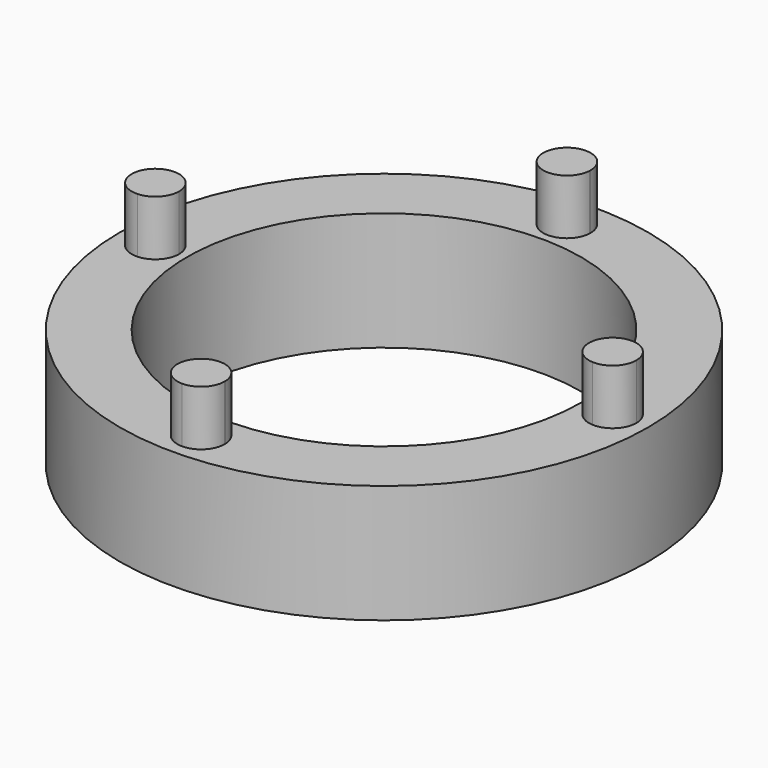
from build123d import *

# Parameters (mm, degrees)
F1_DEPTH = 8.89
F0_R     = 42.545
F0_R_2   = 31.75
F2_DEPTH = 19.05


with BuildPart() as f1:
    # F0 (on Top) → F1 (new body)
    with BuildSketch(Plane.XY):
        with BuildLine():
            ThreePointArc((3.81, 36.83), (2.6940768363, 39.5240768363), (0, 40.64))
            ThreePointArc((0, 40.64), (-2.7628728489, 39.4534773909), (-3.8048999754, 36.6329310345))
            ThreePointArc((-3.8048999754, 36.6329310345), (0, 36.83), (3.8048999754, 36.6329310345))
            ThreePointArc((3.8048999754, 36.6329310345), (3.8087247804, 36.7314325264), (3.81, 36.83))
        make_face()
        with BuildLine():
            ThreePointArc((3.8048999754, 36.6329310345), (0, 36.83), (-3.8048999754, 36.6329310345))
            ThreePointArc((-3.8048999754, 36.6329310345), (0, 33.02), (3.8048999754, 36.6329310345))
        make_face()
    extrude(amount=F1_DEPTH)


with BuildPart() as f1b:
    # F0 (on Top) → F1, piece 2 (new body)
    with BuildSketch(Plane.XY):
        with BuildLine():
            ThreePointArc((-33.02, 0), (-34.0671271511, 2.6234773909), (-36.6329310345, 3.8048999754))
            ThreePointArc((-36.6329310345, 3.8048999754), (-36.83, 0), (-36.6329310345, -3.8048999754))
            ThreePointArc((-36.6329310345, -3.8048999754), (-34.0671271511, -2.6234773909), (-33.02, 0))
        make_face()
        with BuildLine():
            ThreePointArc((-36.6329310345, 3.8048999754), (-39.4534773924, 2.7628728475), (-40.64, -4.1e-09))
            ThreePointArc((-40.64, -4.1e-09), (-39.4534773894, -2.7628728503), (-36.6329310345, -3.8048999754))
            ThreePointArc((-36.6329310345, -3.8048999754), (-36.83, 0), (-36.6329310345, 3.8048999754))
        make_face()
    extrude(amount=F1_DEPTH)


with BuildPart() as f1c:
    # F0 (on Top) → F1, piece 3 (new body)
    with BuildSketch(Plane.XY):
        with BuildLine():
            ThreePointArc((36.83, 0), (36.7806997622, 1.905), (36.6329310345, 3.8048999754))
            ThreePointArc((36.6329310345, 3.8048999754), (33.02, 0), (36.6329310345, -3.8048999754))
            ThreePointArc((36.6329310345, -3.8048999754), (36.7806997622, -1.905), (36.83, 0))
        make_face()
        with BuildLine():
            ThreePointArc((36.6329310345, -3.8048999754), (39.4534773909, -2.7628728489), (40.64, 0))
            ThreePointArc((40.64, 0), (39.4534773909, 2.7628728489), (36.6329310345, 3.8048999754))
            ThreePointArc((36.6329310345, 3.8048999754), (36.7806997622, 1.905), (36.83, 0))
            ThreePointArc((36.83, 0), (36.7806997622, -1.905), (36.6329310345, -3.8048999754))
        make_face()
    extrude(amount=F1_DEPTH)


with BuildPart() as f1d:
    # F0 (on Top) → F1, piece 4 (new body)
    with BuildSketch(Plane.XY):
        with BuildLine():
            ThreePointArc((3.8048999754, -36.6329310345), (0, -33.02), (-3.8048999754, -36.6329310345))
            ThreePointArc((-3.8048999754, -36.6329310345), (0, -36.83), (3.8048999754, -36.6329310345))
        make_face()
        with BuildLine():
            ThreePointArc((-3.8048999754, -36.6329310345), (-2.7628728415, -39.4534773987), (2.15e-08, -40.64))
            ThreePointArc((2.15e-08, -40.64), (2.6940768439, -39.5240768287), (3.81, -36.83))
            ThreePointArc((3.81, -36.83), (3.8087247804, -36.7314325264), (3.8048999754, -36.6329310345))
            ThreePointArc((3.8048999754, -36.6329310345), (0, -36.83), (-3.8048999754, -36.6329310345))
        make_face()
    extrude(amount=F1_DEPTH)


with BuildPart() as f2:
    # F0 (on Top) → F2 (new body)
    with BuildSketch(Plane.XY):
        Circle(F0_R)
        with BuildLine():
            ThreePointArc((0, 40.64), (28.7368195874, 28.7368195874), (40.64, 0))
            ThreePointArc((40.64, 0), (28.736819595, -28.7368195798), (2.15e-08, -40.64))
            ThreePointArc((2.15e-08, -40.64), (-28.7368195784, -28.7368195965), (-40.64, -4.1e-09))
            ThreePointArc((-40.64, -4.1e-09), (-28.7368195889, 28.736819586), (0, 40.64))
        make_face(mode=Mode.SUBTRACT)
        with BuildLine():
            ThreePointArc((36.6329310345, -3.8048999754), (33.02, 0), (36.6329310345, 3.8048999754))
            ThreePointArc((36.6329310345, 3.8048999754), (26.0427427511, 26.0427427511), (3.8048999754, 36.6329310345))
            ThreePointArc((3.8048999754, 36.6329310345), (0, 33.02), (-3.8048999754, 36.6329310345))
            ThreePointArc((-3.8048999754, 36.6329310345), (-26.0427427511, 26.0427427511), (-36.6329310345, 3.8048999754))
            ThreePointArc((-36.6329310345, 3.8048999754), (-34.0671271511, 2.6234773909), (-33.02, 0))
            ThreePointArc((-33.02, 0), (-34.0671271511, -2.6234773909), (-36.6329310345, -3.8048999754))
            ThreePointArc((-36.6329310345, -3.8048999754), (-26.0427427511, -26.0427427511), (-3.8048999754, -36.6329310345))
            ThreePointArc((-3.8048999754, -36.6329310345), (0, -33.02), (3.8048999754, -36.6329310345))
            ThreePointArc((3.8048999754, -36.6329310345), (26.0427427511, -26.0427427511), (36.6329310345, -3.8048999754))
        make_face()
        Circle(F0_R_2, mode=Mode.SUBTRACT)
        with BuildLine():
            ThreePointArc((36.6329310345, 3.8048999754), (39.4534773909, 2.7628728489), (40.64, 0))
            ThreePointArc((40.64, 0), (28.7368195874, 28.7368195874), (0, 40.64))
            ThreePointArc((0, 40.64), (2.6940768363, 39.5240768363), (3.81, 36.83))
            ThreePointArc((3.81, 36.83), (3.8087247804, 36.7314325264), (3.8048999754, 36.6329310345))
            ThreePointArc((3.8048999754, 36.6329310345), (26.0427427511, 26.0427427511), (36.6329310345, 3.8048999754))
        make_face()
        with BuildLine():
            ThreePointArc((2.15e-08, -40.64), (28.736819595, -28.7368195798), (40.64, 0))
            ThreePointArc((40.64, 0), (39.4534773909, -2.7628728489), (36.6329310345, -3.8048999754))
            ThreePointArc((36.6329310345, -3.8048999754), (26.0427427511, -26.0427427511), (3.8048999754, -36.6329310345))
            ThreePointArc((3.8048999754, -36.6329310345), (3.8087247804, -36.7314325264), (3.81, -36.83))
            ThreePointArc((3.81, -36.83), (2.6940768439, -39.5240768287), (2.15e-08, -40.64))
        make_face()
        with BuildLine():
            ThreePointArc((-3.8048999754, 36.6329310345), (-2.7628728489, 39.4534773909), (0, 40.64))
            ThreePointArc((0, 40.64), (-28.7368195889, 28.736819586), (-40.64, -4.1e-09))
            ThreePointArc((-40.64, -4.1e-09), (-39.4534773924, 2.7628728475), (-36.6329310345, 3.8048999754))
            ThreePointArc((-36.6329310345, 3.8048999754), (-26.0427427511, 26.0427427511), (-3.8048999754, 36.6329310345))
        make_face()
        with BuildLine():
            ThreePointArc((-40.64, -4.1e-09), (-28.7368195784, -28.7368195965), (2.15e-08, -40.64))
            ThreePointArc((2.15e-08, -40.64), (-2.7628728415, -39.4534773987), (-3.8048999754, -36.6329310345))
            ThreePointArc((-3.8048999754, -36.6329310345), (-26.0427427511, -26.0427427511), (-36.6329310345, -3.8048999754))
            ThreePointArc((-36.6329310345, -3.8048999754), (-39.4534773894, -2.7628728503), (-40.64, -4.1e-09))
        make_face()
        with BuildLine():
            ThreePointArc((36.6329310345, -3.8048999754), (39.4534773909, -2.7628728489), (40.64, 0))
            ThreePointArc((40.64, 0), (39.4534773909, 2.7628728489), (36.6329310345, 3.8048999754))
            ThreePointArc((36.6329310345, 3.8048999754), (36.7806997622, 1.905), (36.83, 0))
            ThreePointArc((36.83, 0), (36.7806997622, -1.905), (36.6329310345, -3.8048999754))
        make_face()
        with BuildLine():
            ThreePointArc((3.81, 36.83), (2.6940768363, 39.5240768363), (0, 40.64))
            ThreePointArc((0, 40.64), (-2.7628728489, 39.4534773909), (-3.8048999754, 36.6329310345))
            ThreePointArc((-3.8048999754, 36.6329310345), (0, 36.83), (3.8048999754, 36.6329310345))
            ThreePointArc((3.8048999754, 36.6329310345), (3.8087247804, 36.7314325264), (3.81, 36.83))
        make_face()
        with BuildLine():
            ThreePointArc((-3.8048999754, -36.6329310345), (-2.7628728415, -39.4534773987), (2.15e-08, -40.64))
            ThreePointArc((2.15e-08, -40.64), (2.6940768439, -39.5240768287), (3.81, -36.83))
            ThreePointArc((3.81, -36.83), (3.8087247804, -36.7314325264), (3.8048999754, -36.6329310345))
            ThreePointArc((3.8048999754, -36.6329310345), (0, -36.83), (-3.8048999754, -36.6329310345))
        make_face()
        with BuildLine():
            ThreePointArc((-36.6329310345, 3.8048999754), (-39.4534773924, 2.7628728475), (-40.64, -4.1e-09))
            ThreePointArc((-40.64, -4.1e-09), (-39.4534773894, -2.7628728503), (-36.6329310345, -3.8048999754))
            ThreePointArc((-36.6329310345, -3.8048999754), (-36.83, 0), (-36.6329310345, 3.8048999754))
        make_face()
        with BuildLine():
            ThreePointArc((36.83, 0), (36.7806997622, 1.905), (36.6329310345, 3.8048999754))
            ThreePointArc((36.6329310345, 3.8048999754), (33.02, 0), (36.6329310345, -3.8048999754))
            ThreePointArc((36.6329310345, -3.8048999754), (36.7806997622, -1.905), (36.83, 0))
        make_face()
        with BuildLine():
            ThreePointArc((3.8048999754, 36.6329310345), (0, 36.83), (-3.8048999754, 36.6329310345))
            ThreePointArc((-3.8048999754, 36.6329310345), (0, 33.02), (3.8048999754, 36.6329310345))
        make_face()
        with BuildLine():
            ThreePointArc((3.8048999754, -36.6329310345), (0, -33.02), (-3.8048999754, -36.6329310345))
            ThreePointArc((-3.8048999754, -36.6329310345), (0, -36.83), (3.8048999754, -36.6329310345))
        make_face()
        with BuildLine():
            ThreePointArc((-33.02, 0), (-34.0671271511, 2.6234773909), (-36.6329310345, 3.8048999754))
            ThreePointArc((-36.6329310345, 3.8048999754), (-36.83, 0), (-36.6329310345, -3.8048999754))
            ThreePointArc((-36.6329310345, -3.8048999754), (-34.0671271511, -2.6234773909), (-33.02, 0))
        make_face()
    extrude(amount=-F2_DEPTH)


solid = Compound([f1.part, f1b.part, f1c.part, f1d.part, f2.part])
